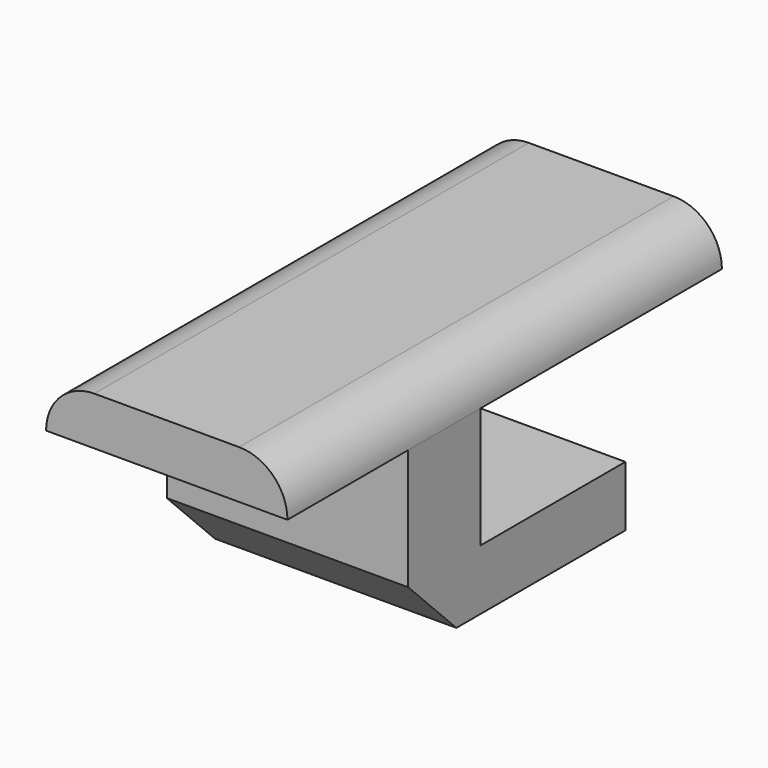
from build123d import *

# Parameters (mm, degrees)
F0_W     = 40
F0_H     = 90
F1_DEPTH = 8
F2_W     = 40
F2_H     = 15
F3_DEPTH = 30
F4_W     = 40
F4_H     = 10
F5_DEPTH = 30
F6_R     = 7.99999
F7_SIZE2 = 10
F7_SIZE  = 10


# Not quite as in the source:
# - a fillet or chamfer is up to 0.001 mm smaller than in the source, because OpenCascade refuses the exact size


with BuildPart() as f1:
    # F0 (on Top) → F1 (new body)
    with BuildSketch(Plane.XY):
        with Locations((-20, 7.0996452868)):
            Rectangle(F0_W, F0_H)
    extrude(amount=F1_DEPTH)

    # F2 (on face) → F3 (join)
    with BuildSketch(Plane(origin=(0, 0, 0), x_dir=(1, 0, 0), z_dir=(0, 0, -1))):
        with Locations((-20, 5.4003547132)):
            Rectangle(F2_W, F2_H)
    extrude(amount=F3_DEPTH)

    # F4 (on face) → F5 (join)
    with BuildSketch(Plane(origin=(0, 2.0996452868, 0), x_dir=(-1, 0, 0), z_dir=(0, 1, 0))):
        with Locations((20, -25)):
            Rectangle(F4_W, F4_H)
    extrude(amount=F5_DEPTH)

    # F6 (radius 8 in the source; OpenCascade refuses exactly that, so slightly less here)
    f6_edges = [f1.edges().sort_by_distance(p)[0] for p in [
        (0, 7.099645, 8),
        (-40, 7.099645, 8),
    ]]
    fillet(f6_edges, radius=F6_R)

    # F7
    f7_edges = [f1.edges().sort_by_distance(p)[0] for p in [
        (-20, -12.900355, -30),
    ]]
    chamfer(f7_edges, length=F7_SIZE, length2=F7_SIZE2)


solid = f1.part
